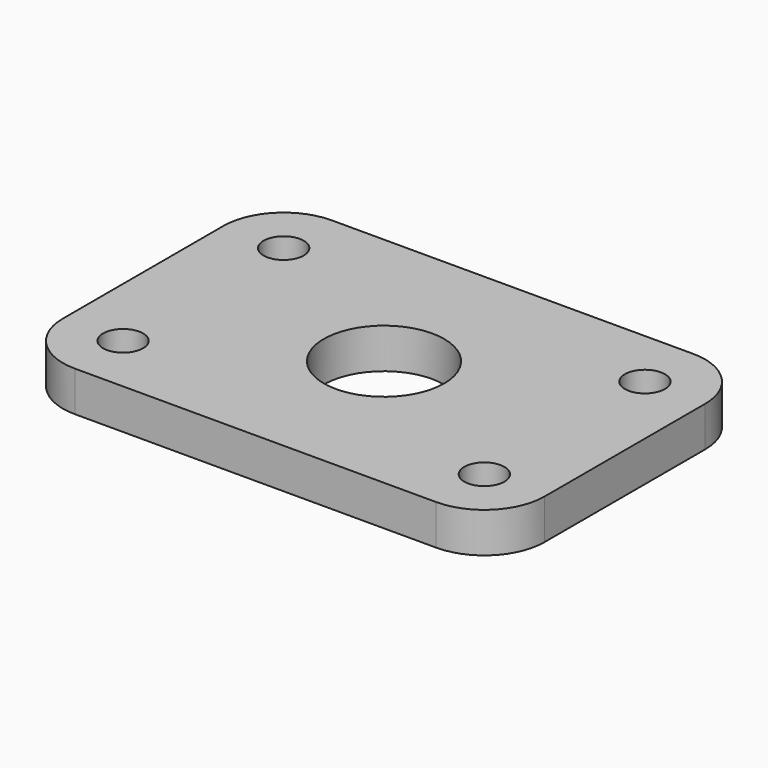
from build123d import *

# Parameters (mm, degrees)
F0_R     = 6.35
F0_R_2   = 19.05
F1_DEPTH = 12.7


# Not quite as in the source:
# - a feature names something its author has since deleted; it is built from what else it names


with BuildPart() as f1:
    # F0 (on Top) → F1 (new body)
    with BuildSketch(Plane.XY):
        with BuildLine():
            ThreePointArc((76.2, 31.75), (70.6203841816, 45.2203841816), (57.15, 50.8))
            Line((57.15, 50.8), (-57.15, 50.8))
            ThreePointArc((-57.15, 50.8), (-70.6203841816, 45.2203841816), (-76.2, 31.75))
            Line((-76.2, 31.75), (-76.2, -31.75))
            ThreePointArc((-76.2, -31.75), (-70.6203841816, -45.2203841816), (-57.15, -50.8))
            Line((-57.15, -50.8), (57.15, -50.8))
            ThreePointArc((57.15, -50.8), (70.6203841816, -45.2203841816), (76.2, -31.75))
            Line((76.2, -31.75), (76.2, 31.75))
        make_face()
        with Locations((-57.15, -31.75)):
            Circle(F0_R, mode=Mode.SUBTRACT)
        with Locations((57.15, -31.75)):
            Circle(F0_R, mode=Mode.SUBTRACT)
        Circle(F0_R_2, mode=Mode.SUBTRACT)
        with Locations((-57.15, 31.75)):
            Circle(F0_R, mode=Mode.SUBTRACT)
        with Locations((57.15, 31.75)):
            Circle(F0_R, mode=Mode.SUBTRACT)
    extrude(amount=F1_DEPTH)


solid = f1.part
